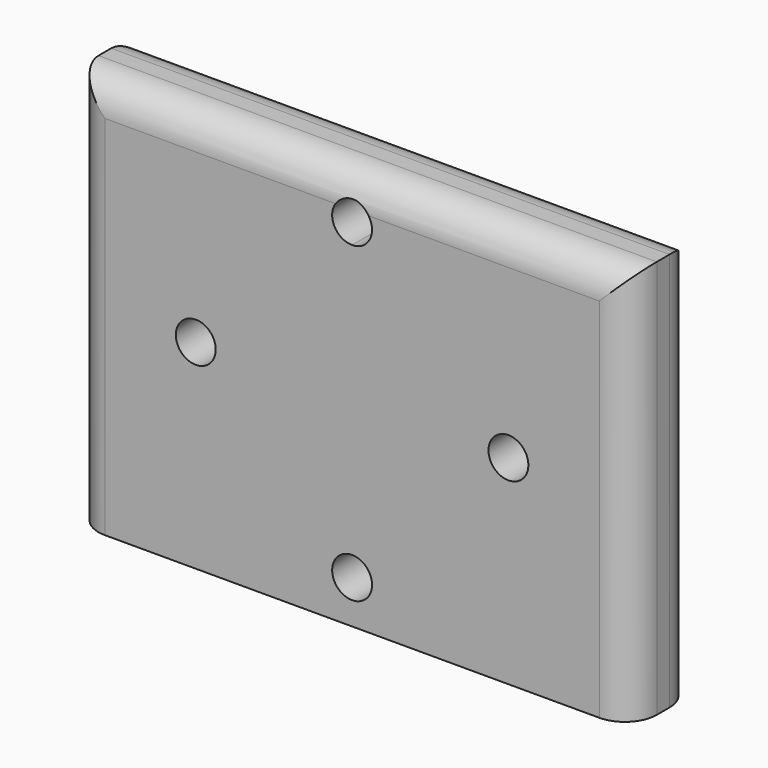
from build123d import *

# Parameters (mm, degrees)
F0_W        = 88.9
F0_H        = 63.5
F0_R        = 3.175
F1_DEPTH    = 6.35
F2_R        = 3.81
F3_DEPTH    = 25.4
F4_T1_DEPTH = 88.9
F4_T3_DEPTH = 114.3


# Not quite as in the source:
# - a fillet or chamfer that OpenCascade refuses, or shapes differently, is made with other operations: its cross-section is extruded or revolved along the edge and cut away or added


with BuildPart() as f1:
    # F0 (on Front) → F1 (new body, symmetric)
    with BuildSketch(Plane.XZ):
        Rectangle(F0_W, F0_H)
        with Locations((0, -24.892)):
            Circle(F0_R, mode=Mode.SUBTRACT)
        with BuildLine():
            ThreePointArc((-21.717, 0), (-24.892, -3.175), (-28.067, 0))
            ThreePointArc((-28.067, 0), (-24.892, 3.175), (-21.717, 0))
        make_face(mode=Mode.SUBTRACT)
        with Locations((24.892, 0)):
            Circle(F0_R, mode=Mode.SUBTRACT)
        with BuildLine():
            ThreePointArc((0, 21.717), (-3.175, 24.892), (0, 28.067))
            ThreePointArc((0, 28.067), (2.2450640303, 27.1370640303), (3.175, 24.892))
            ThreePointArc((3.175, 24.892), (2.2450640303, 22.6469359697), (0, 21.717))
        make_face(mode=Mode.SUBTRACT)
    extrude(amount=F1_DEPTH, both=True)

    # F2 (on face) → F3 (cut)
    with BuildSketch(Plane(origin=(0, 0, -31.75), x_dir=(1, 0, 0), z_dir=(0, 0, -1))):
        with Locations((-25.4, 0)):
            Circle(F2_R)
        with BuildLine():
            ThreePointArc((29.21, 0), (25.4, 3.81), (21.59, 0))
            ThreePointArc((21.59, 0), (25.4, -3.81), (29.21, 0))
        make_face()
    extrude(amount=-F3_DEPTH, mode=Mode.SUBTRACT)

    # F4: fillet of radius 5.08 on 6 edges, made by hand

    # F4_s2 → F4_t1 (cut)
    with BuildSketch(Plane.XY.offset(-44.45)):
        with BuildLine():
            ThreePointArc((-44.45, -1.27), (-42.9621024484, -4.8621024484), (-39.37, -6.35))
            Line((-39.37, -6.35), (-44.45, -6.35))
            Line((-44.45, -6.35), (-44.45, -1.27))
        make_face()
        with BuildLine():
            ThreePointArc((44.45, -1.27), (42.9621024484, -4.8621024484), (39.37, -6.35))
            Line((39.37, -6.35), (44.45, -6.35))
            Line((44.45, -6.35), (44.45, -1.27))
        make_face()
        with BuildLine():
            ThreePointArc((39.37, 6.35), (42.9621024484, 4.8621024484), (44.45, 1.27))
            Line((44.45, 1.27), (44.45, 6.35))
            Line((44.45, 6.35), (39.37, 6.35))
        make_face()
        with BuildLine():
            ThreePointArc((-39.37, 6.35), (-42.9621024484, 4.8621024484), (-44.45, 1.27))
            Line((-44.45, 1.27), (-44.45, 6.35))
            Line((-44.45, 6.35), (-39.37, 6.35))
        make_face()
    extrude(amount=F4_T1_DEPTH, mode=Mode.SUBTRACT)

    # F4_s4 → F4_t3 (cut)
    with BuildSketch(Plane.YZ.offset(-57.15)):
        with BuildLine():
            ThreePointArc((-6.35, 26.67), (-4.8621024484, 30.2621024484), (-1.27, 31.75))
            Line((-1.27, 31.75), (-6.35, 31.75))
            Line((-6.35, 31.75), (-6.35, 26.67))
        make_face()
        with BuildLine():
            ThreePointArc((6.35, 26.67), (4.8621024484, 30.2621024484), (1.27, 31.75))
            Line((1.27, 31.75), (6.35, 31.75))
            Line((6.35, 31.75), (6.35, 26.67))
        make_face()
    extrude(amount=F4_T3_DEPTH, mode=Mode.SUBTRACT)


solid = f1.part
